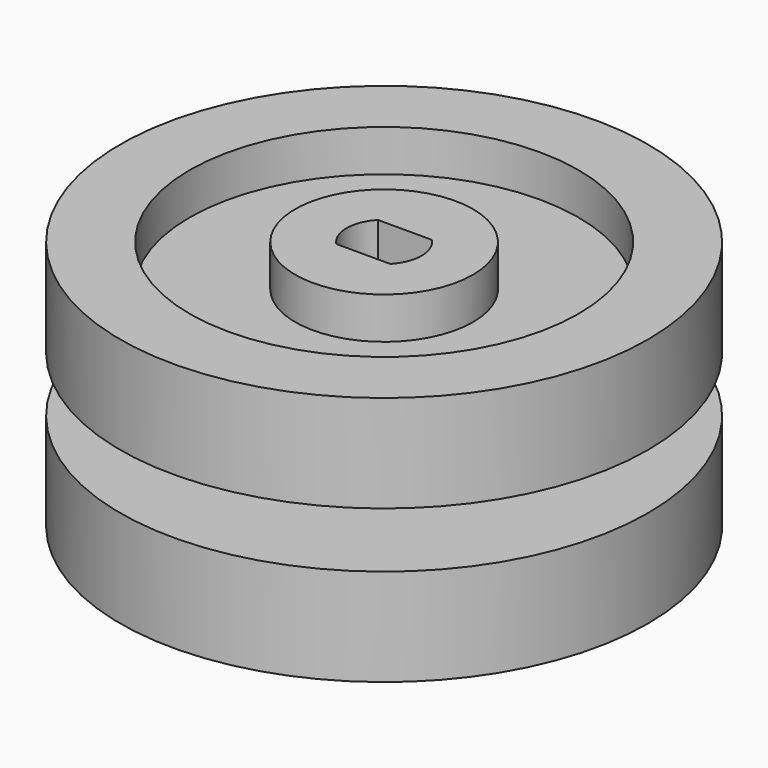
from build123d import *

# Parameters (mm, degrees)
F0_R      = 19
F1_DEPTH  = 7
F2_R      = 11.25
F3_DEPTH  = 2
F4_R      = 14
F4_R_2    = 6.4
F5_DEPTH  = 3
F8_DEPTH  = 6
F9_R      = 1.5
F10_DEPTH = 12


# Not quite as in the source:
# - a feature names something its author has since deleted; it is built from what else it names


with BuildPart() as f1:
    # F0 (on Top) → F1 (new body)
    with BuildSketch(Plane.XY):
        Circle(F0_R)
    extrude(amount=F1_DEPTH)

    # F2 (on face) → F3 (join)
    with BuildSketch(Plane(origin=(0, 0, 0), x_dir=(1, 0, 0), z_dir=(0, 0, -1))):
        Circle(F2_R)
    extrude(amount=F3_DEPTH)

    # F4 (on face) → F5 (cut)
    with BuildSketch(Plane.XY.offset(7)):
        Circle(F4_R)
        Circle(F4_R_2, mode=Mode.SUBTRACT)
    extrude(amount=-F5_DEPTH, mode=Mode.SUBTRACT)

    # F6: F1 across face


with BuildPart() as f1_1:
    add(f1.part)
    add(f1.part.mirror(Plane(origin=(0, 0, -2), x_dir=(1, 0, 0), z_dir=(0, 0, -1))))

    # F7 (on face) → F8 (cut)
    with BuildSketch(Plane.XY.offset(7)):
        with BuildLine():
            Line((1.942775077, 1.875), (-1.942775077, 1.875))
            ThreePointArc((-1.942775077, 1.875), (-2.7, 0), (-1.942775077, -1.875))
            Line((-1.942775077, -1.875), (1.942775077, -1.875))
            ThreePointArc((1.942775077, -1.875), (2.7, 0), (1.942775077, 1.875))
        make_face()
    extrude(amount=-F8_DEPTH, mode=Mode.SUBTRACT)

    # F9 (on face) → F10 (cut, through all)
    with BuildSketch(Plane(origin=(0, 0, -11), x_dir=(1, 0, 0), z_dir=(0, 0, -1))):
        Circle(F9_R)
    extrude(amount=-F10_DEPTH, mode=Mode.SUBTRACT)


solid = f1_1.part
